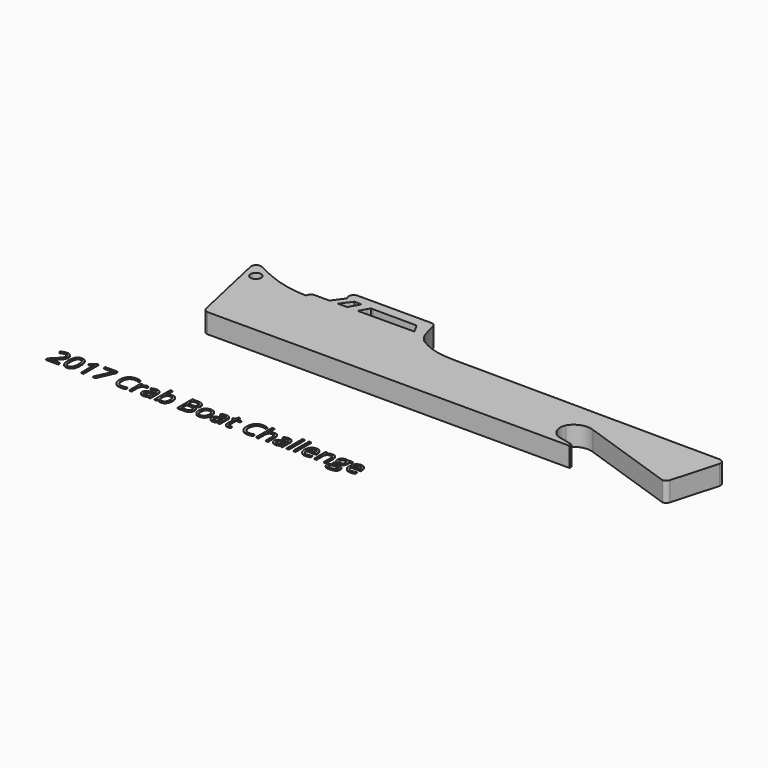
from build123d import *

# Parameters (mm, degrees)
F0_R         = 1.7144531012
F2_DEPTH     = 6.35
F1_TEXT_SIZE = 8.4224451373
F3_DEPTH     = 0.254


# Not quite as in the source:
# - Text() gives the source's letters only with a copy of the font that has no kerning and outlines rounded to 1/6400 em; it was checked with that copy


with BuildPart() as f2:
    # F0 (on Top) → F2 (new body)
    with BuildSketch(Plane.XY):
        with BuildLine():
            ThreePointArc((-82.6578963548, 16.6351178779), (-84.3524050739, 16.4782032173), (-84.9313041555, 14.8779351576))
            Line((-84.9313041555, 14.8779351576), (-79.3758570051, -10.1331158304))
            ThreePointArc((-79.3758570051, -10.1331158304), (-78.8195291366, -11.0271579858), (-77.826126409, -11.3763901348))
            Line((-77.826126409, -11.3763901348), (38.8641767204, -11.3763901348))
            Line((38.8641767204, -11.3763901348), (39.6109595895, -11.3763901348))
            Line((39.6109595895, -11.3763901348), (39.6109595895, -10.4980878532))
            Line((39.6109595895, -10.4980878532), (34.6225580335, -9.3062752848))
            ThreePointArc((34.6225580335, -9.3062752848), (31.8870143048, -6.8536670921), (31.866350634, -3.1796965627))
            ThreePointArc((31.866350634, -3.1796965627), (34.9358763859, -0.7250128646), (38.8641767204, -0.8511749911))
            Line((38.8641767204, -0.8511749911), (69.7269539483, -11.3763901348))
            ThreePointArc((69.7269539483, -11.3763901348), (70.6839738092, -11.0554876382), (71.254083355, -10.2225167311))
            Line((71.254083355, -10.2225167311), (75.4562824837, 4.5766259358))
            ThreePointArc((75.4562824837, 4.5766259358), (75.19873204, 5.9633136564), (73.9390647666, 6.5977215896))
            Line((73.9390647666, 6.5977215896), (-11.3526463776, 7.130257934))
            add(Edge.make_bspline(
                [(-12.8668220646, 7.1397120014), (-12.372094858, 7.1289012328), (-11.8671693523, 7.1257865528), (-11.3526463776, 7.130257934)],
                knots=[0.4231373007, 0.4231373007, 0.4231373007, 0.4231373007, 0.4697559219, 0.4697559219, 0.4697559219, 0.4697559219], degree=3))
            add(Edge.make_bspline(
                [(-24.3954672646, 10.0651517198), (-21.0074985022, 7.9699973196), (-17.3572494873, 7.2378367273), (-12.8668220646, 7.1397120014)],
                knots=[0, 0, 0, 0, 0.4231373007, 0.4231373007, 0.4231373007, 0.4231373007], degree=3))
            add(Edge.make_bspline(
                [(-28.386289363, 18.2088658517), (-27.5680035145, 14.8439996122), (-27.0323755451, 11.694124655), (-24.3954672646, 10.0651517198)],
                knots=[0.0520925717, 0.0520925717, 0.0520925717, 0.0520925717, 0.4883396262, 0.4883396262, 0.4883396262, 0.4883396262], degree=3))
            ThreePointArc((-28.386289363, 18.2088658517), (-28.9478512317, 19.0818737964), (-29.9288322239, 19.4212421755))
            Line((-29.9288322239, 19.4212421755), (-46.1653646044, 19.4212421755))
            add(Edge.make_bspline(
                [(-46.1891002262, 16.0552153603), (-45.8007262833, 16.4726439919), (-45.170890508, 17.5631013885), (-45.5943751344, 18.7109734238), (-46.1653646044, 19.4212421755)],
                knots=[0.6051427411, 0.6051427411, 0.6051427411, 0.6051427411, 0.646637232, 0.7098733844, 0.7098733844, 0.7098733844, 0.7098733844], degree=3))
            Line((-46.1891002262, 16.0552153603), (-31.8741314113, 15.990441665))
            Line((-31.8741314113, 15.990441665), (-30.251037274, 13.0147728891))
            Line((-30.251037274, 13.0147728891), (-48.5709768547, 12.9124532739))
            Line((-48.5709768547, 12.9124532739), (-47.355101634, 15.0968942509))
            add(Edge.make_bspline(
                [(-51.8151050758, 13.1146471412), (-50.0243845057, 13.6812317066), (-48.4772240612, 14.3547573158), (-47.355101634, 15.0968942509)],
                knots=[0.493608635, 0.493608635, 0.493608635, 0.493608635, 0.5723926752, 0.5723926752, 0.5723926752, 0.5723926752], degree=3))
            Line((-51.8151050758, 13.1146471412), (-51.9381151423, 12.8936473007))
            Line((-51.9381151423, 12.8936473007), (-52.5564191218, 12.89019398))
            add(Edge.make_bspline(
                [(-64.1152808122, 11.3057810813), (-60.2915866445, 11.268947734), (-56.0377535586, 11.8817545575), (-52.5564191218, 12.89019398)],
                knots=[0.3349455176, 0.3349455176, 0.3349455176, 0.3349455176, 0.4829274162, 0.4829274162, 0.4829274162, 0.4829274162], degree=3))
            add(Edge.make_bspline(
                [(-82.6578963548, 16.6351178779), (-77.1639177835, 13.8212551878), (-71.4257434064, 11.3762021967), (-64.1152808122, 11.3057810813)],
                knots=[0.0520211814, 0.0520211814, 0.0520211814, 0.0520211814, 0.3349455176, 0.3349455176, 0.3349455176, 0.3349455176], degree=3))
        make_face()
        with Locations((-80.698594451, 11.7666525766)):
            Circle(F0_R, mode=Mode.SUBTRACT)
        with BuildLine():
            Line((-63.9558078515, 11.7798734638), (-64.1152808122, 11.3057810813))
            add(Edge.make_bspline(
                [(-64.1152808122, 11.3057810813), (-60.2915866445, 11.268947734), (-56.0377535586, 11.8817545575), (-52.5564191218, 12.89019398)],
                knots=[0.3349455176, 0.3349455176, 0.3349455176, 0.3349455176, 0.4829274162, 0.4829274162, 0.4829274162, 0.4829274162], degree=3))
            Line((-52.5564191218, 12.89019398), (-54.9355708063, 12.8769060604))
            Line((-54.9355708063, 12.8769060604), (-52.3232373834, 16.3812569725))
            Line((-52.3232373834, 16.3812569725), (-50.0494301007, 16.2868581559))
            Line((-50.0494301007, 16.2868581559), (-51.8151050758, 13.1146471412))
            add(Edge.make_bspline(
                [(-51.8151050758, 13.1146471412), (-50.0243845057, 13.6812317066), (-48.4772240612, 14.3547573158), (-47.355101634, 15.0968942509)],
                knots=[0.493608635, 0.493608635, 0.493608635, 0.493608635, 0.5723926752, 0.5723926752, 0.5723926752, 0.5723926752], degree=3))
            Line((-47.355101634, 15.0968942509), (-46.8201041222, 16.0580705851))
            Line((-46.8201041222, 16.0580705851), (-46.1891002262, 16.0552153603))
            add(Edge.make_bspline(
                [(-46.1891002262, 16.0552153603), (-45.8007262833, 16.4726439919), (-45.170890508, 17.5631013885), (-45.5943751344, 18.7109734238), (-46.1653646044, 19.4212421755)],
                knots=[0.6051427411, 0.6051427411, 0.6051427411, 0.6051427411, 0.646637232, 0.7098733844, 0.7098733844, 0.7098733844, 0.7098733844], degree=3))
            Line((-46.1653646044, 19.4212421755), (-53.7738942729, 19.4212421755))
            ThreePointArc((-53.7738942729, 19.4212421755), (-55.116215914, 18.6812850133), (-55.2071857286, 17.1512234189))
            Line((-55.2071857286, 17.1512234189), (-54.9355708063, 16.5808312595))
            Line((-54.9355708063, 16.5808312595), (-57.7083528042, 12.8612443805))
            Line((-57.7083528042, 12.8612443805), (-62.4511518772, 12.8612443805))
            ThreePointArc((-62.4511518772, 12.8612443805), (-63.3776172922, 12.5628596138), (-63.9558078515, 11.7798734638))
        make_face()
    extrude(amount=F2_DEPTH)


with BuildPart() as f3:
    # F1 (on Top) → F3 (new body)
    with BuildSketch(Plane.XY):
        with Locations((-101.39439539, -47.9813217146)):
            Text('2017 Crab Boat Challenge', F1_TEXT_SIZE, font='Open Sans', text_align=(TextAlign.LEFT, TextAlign.BOTTOM))
    extrude(amount=F3_DEPTH)


solid = Compound([f2.part, f3.part])
